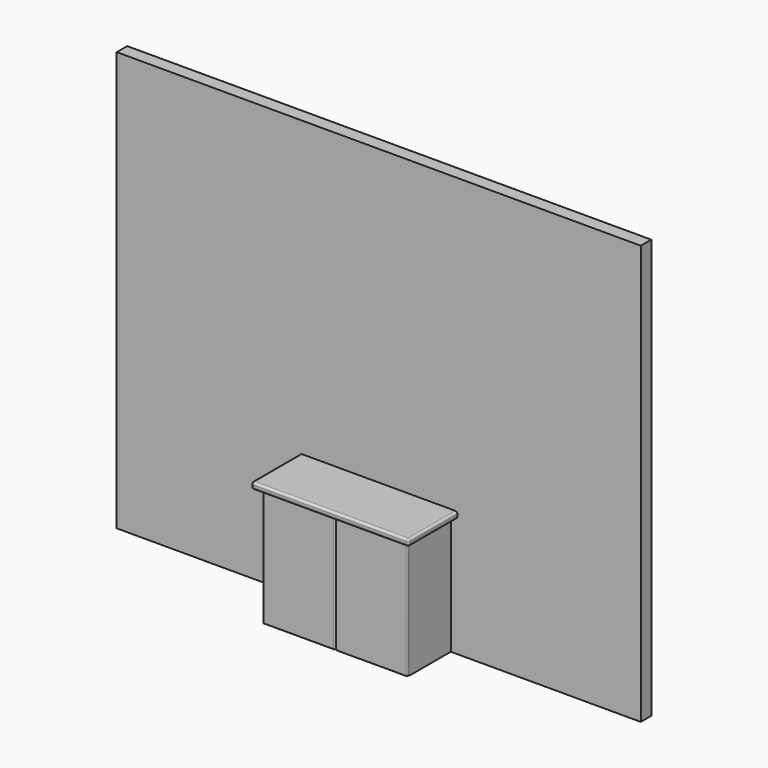
from build123d import *

# Parameters (mm, degrees)
F0_W     = 3048
F0_H     = 2438.4
F1_DEPTH = 76.2
F2_W     = 914.4
F2_H     = 38.1
F3_DEPTH = 355.6
F4_R     = 12.7
F5_R     = 12.7
F7_DEPTH = 692.15
F8_R     = 6.35
F8_2_R   = 6.35
F9_R     = 6.35
F9_2_R   = 6.35


# Not quite as in the source:
# - ends of sketch curves that miss each other by under 0.0002 mm in the source are joined


with BuildPart() as f1:
    # F0 (on Front) → F1 (new body)
    with BuildSketch(Plane.XZ):
        Rectangle(F0_W, F0_H)
    extrude(amount=F1_DEPTH)


with BuildPart() as f3:
    # F2 (on face) → F3 (new body)
    with BuildSketch(Plane.XZ.offset(76.2)):
        with Locations((0, -508)):
            Rectangle(F2_W, F2_H)
    extrude(amount=F3_DEPTH)

    # F4
    f4_edges = [f3.edges().sort_by_distance(p)[0] for p in [
        (457.2, -431.8, -508),
        (-457.2, -431.8, -508),
    ]]
    fillet(f4_edges, radius=F4_R)

    # F5
    f5_edges = [f3.edges().sort_by_distance(p)[0] for p in [
        (457.2, -247.65, -488.95),
        (457.2, -247.65, -527.05),
        (0, -431.8, -488.95),
        (0, -431.8, -527.05),
        (-457.2, -247.65, -488.95),
        (-457.2, -247.65, -527.05),
    ]]
    fillet(f5_edges, radius=F5_R)


with BuildPart() as f7:
    # F6 (on face) → F7 (new body)
    with BuildSketch(Plane(origin=(0, 0, -527.05), x_dir=(1, 0, 0), z_dir=(0, 0, -1))):
        Polygon((-419.1, 379.9533247948), (-419.1, 76.2), (419.1, 76.2), (419.100077045, 378.8828551769), (406.400077045, 378.8828551769), (406.400077045, 88.8998284936), (-406.3999652863, 88.8998284936), (-406.3999652863, 379.9533247948), align=None)
    extrude(amount=F7_DEPTH)


with BuildPart() as f7b:
    # F6 (on face) → F7, piece 2 (new body)
    with BuildSketch(Plane(origin=(0, 0, -527.05), x_dir=(1, 0, 0), z_dir=(0, 0, -1))):
        with BuildLine():
            Line((-419.1, 380.9998109937), (-406.3999652863, 380.9998109937))
            Line((-406.3999652863, 380.9998109937), (-2.349158771, 380.9998109937))
            Line((-2.349158771, 380.9998109937), (-2.349158771, 387.3498109937))
            ThreePointArc((-2.349158771, 387.3498109937), (-4.2090307104, 391.8399390542), (-8.699158771, 393.6998109937))
            Line((-8.699158771, 393.6998109937), (-419.099922955, 393.6998109937))
            Line((-419.099922955, 393.6998109937), (-419.1, 380.9998109937))
        make_face()
    extrude(amount=F7_DEPTH)

    # F8#2
    f8_2_edges = [f7b.edges().sort_by_distance(p)[0] for p in [
        (-213.899541, -393.699811, -1219.2),
        (-419.099923, -393.699811, -873.125),
    ]]
    fillet(f8_2_edges, radius=F8_2_R)

    # F9
    f9_edges = [f7b.edges().sort_by_distance(p)[0] for p in [
        (-210.72456, -393.699811, -527.05),
    ]]
    fillet(f9_edges, radius=F9_R)


with BuildPart() as f7c:
    # F6 (on face) → F7, piece 3 (new body)
    with BuildSketch(Plane(origin=(0, 0, -527.05), x_dir=(1, 0, 0), z_dir=(0, 0, -1))):
        with BuildLine():
            Line((419.100077045, 380.9998109937), (419.100077045, 387.3498109937))
            ThreePointArc((419.100077045, 387.3498109937), (417.2402051055, 391.8399390542), (412.750077045, 393.6998109937))
            Line((412.750077045, 393.6998109937), (8.6992916953, 393.6998109937))
            ThreePointArc((8.6992916953, 393.6998109937), (4.2091636347, 391.8399390542), (2.3492916953, 387.3498109937))
            Line((2.3492916953, 387.3498109937), (2.3492916953, 380.9998109937))
            Line((2.3492916953, 380.9998109937), (406.400077045, 380.9998109937))
            Line((406.400077045, 380.9998109937), (419.100077045, 380.9998109937))
        make_face()
    extrude(amount=F7_DEPTH)

    # F8
    f8_edges = [f7c.edges().sort_by_distance(p)[0] for p in [
        (210.724684, -393.699811, -1219.2),
    ]]
    fillet(f8_edges, radius=F8_R)

    # F9#2
    f9_2_edges = [f7c.edges().sort_by_distance(p)[0] for p in [
        (210.724684, -393.699811, -527.05),
    ]]
    fillet(f9_2_edges, radius=F9_2_R)


solid = Compound([f1.part, f3.part, f7.part, f7b.part, f7c.part])
